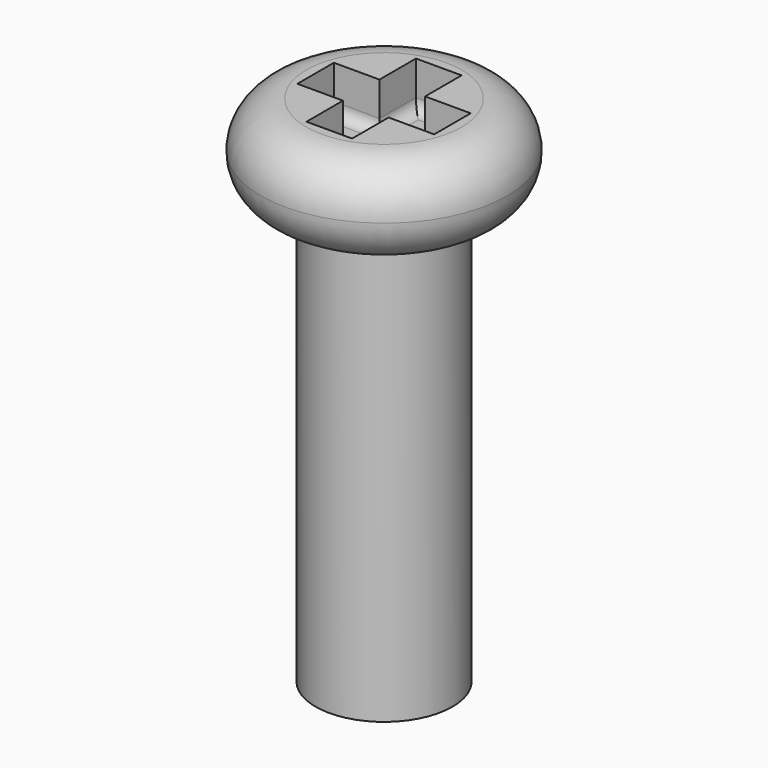
from build123d import *

# Parameters (mm, degrees)
F0_R     = 1.5
F1_DEPTH = 9.25
F2_R     = 2.7
F3_DEPTH = 2
F5_DEPTH = 1
F6_R     = 0.25
F7_R     = 0.99999


# Not quite as in the source:
# - a fillet or chamfer is up to 0.001 mm smaller than in the source, because OpenCascade refuses the exact size


with BuildPart() as f1:
    # F0 (on Top) → F1 (new body)
    with BuildSketch(Plane.XY):
        Circle(F0_R)
    extrude(amount=F1_DEPTH)

    # F2 (on face) → F3 (join)
    with BuildSketch(Plane.XY.offset(9.25)):
        Circle(F2_R)
    extrude(amount=F3_DEPTH)

    # F4 (on face) → F5 (cut)
    with BuildSketch(Plane.XY.offset(11.25)):
        Polygon((0.5, 1.5), (-0.5, 1.5), (-0.5, 0.5), (-1.5, 0.5), (-1.5, -0.5), (-0.5, -0.5), (-0.5, -1.5), (0.5, -1.5), (0.5, -0.5), (1.5, -0.5), (1.5, 0.5), (0.5, 0.5), align=None)
    extrude(amount=-F5_DEPTH, mode=Mode.SUBTRACT)

    # F6
    f6_edges = [f1.edges().sort_by_distance(p)[0] for p in [
        (0, 1.5, 10.25),
        (-0.5, 1, 10.25),
        (-1, 0.5, 10.25),
        (-1.5, 0, 10.25),
        (-1, -0.5, 10.25),
        (-0.5, -1, 10.25),
        (0, -1.5, 10.25),
        (0.5, -1, 10.25),
        (1, -0.5, 10.25),
        (1.5, 0, 10.25),
        (1, 0.5, 10.25),
        (0.5, 1, 10.25),
    ]]
    fillet(f6_edges, radius=F6_R)

    # F7 (radius 1 in the source; OpenCascade refuses exactly that, so slightly less here)
    f7_edges = [f1.edges().sort_by_distance(p)[0] for p in [
        (2.7, 0, 10.25),
        (-2.7, 0, 9.25),
        (-2.7, 0, 11.25),
    ]]
    fillet(f7_edges, radius=F7_R)


solid = f1.part
